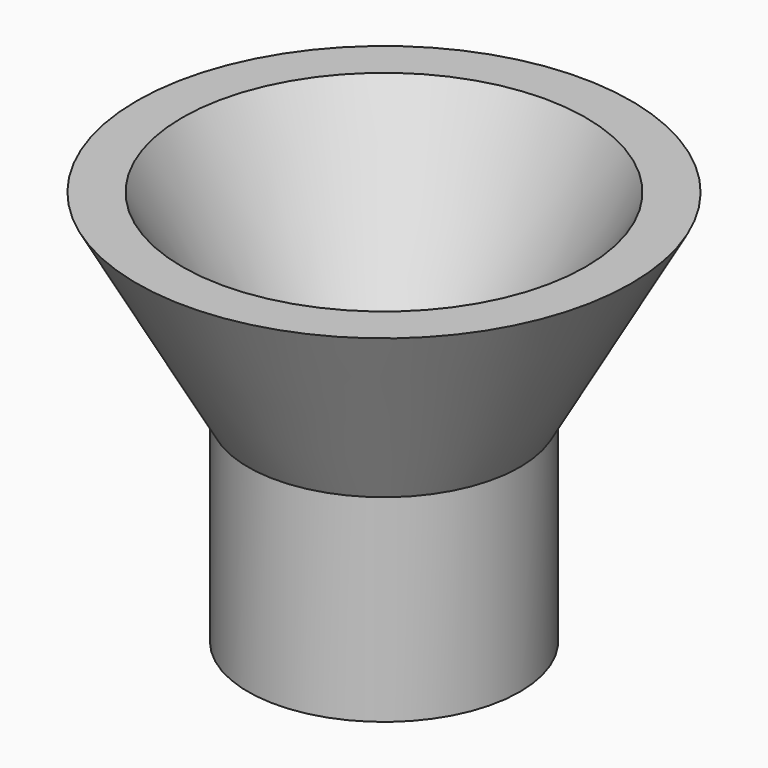
from build123d import *

# Parameters (mm, degrees)
F2_R      = 5
F0_R      = 2.75
F4_R      = 2.75
F6_FACE_R = 2.75
F8_T      = -0.8


with BuildPart() as f6:
    # F2 (on offset) → F6 section 0
    with BuildSketch(Plane.XY.offset(4)):
        Circle(F2_R)
    # F0 (on Top) → F6 section 1
    with BuildSketch(Plane.XY):
        Circle(F0_R)
    loft()

    # F4 (on offset) → F7 section 0
    with BuildSketch(Plane.XY.offset(-4)):
        Circle(F4_R)
    # F6_face (on face) → F7 section 1
    with BuildSketch(Plane(origin=(0, 0, 0), x_dir=(1, 0, 0), z_dir=(0, 0, -1))):
        Circle(F6_FACE_R)
    loft()

    # F8
    f8_openings = [f6.faces().sort_by_distance(p)[0] for p in [
        (0, 0, 4),
        (0, 0, -4),
    ]]
    offset(amount=F8_T, openings=f8_openings, kind=Kind.INTERSECTION)


solid = f6.part
